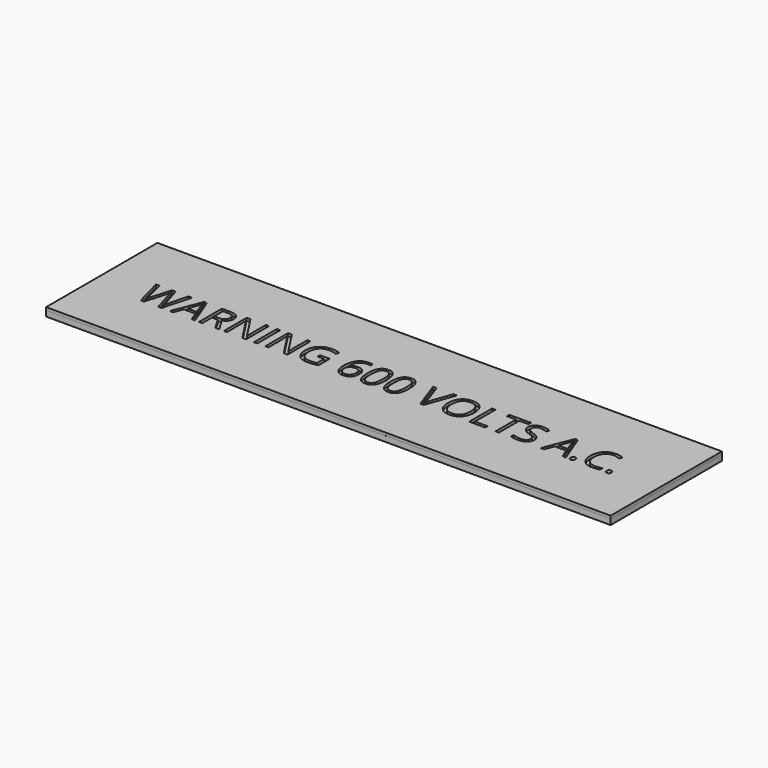
from build123d import *

# Parameters (mm, degrees)
F0_W         = 203.2
F0_H         = 50.08
F1_DEPTH     = 2
F2_DEPTH     = 1
F3_TEXT_SIZE = 14.4258524236
F4_DEPTH     = 1.1


# Not quite as in the source:
# - Text() gives the source's letters only with a copy of the font that has no kerning and outlines rounded to 1/6400 em; it was checked with that copy


with BuildPart() as f1:
    # F0 (on Top) → F1 (new body)
    with BuildSketch(Plane.XY):
        with Locations((75.894802174, 15.1347585702)):
            Rectangle(F0_W, F0_H)
    extrude(amount=F1_DEPTH)


with BuildPart() as f2:
    # F2 (new): a face of the model
    f2_faces = [f1.part.faces().sort_by_distance(p)[0] for p in [
        (75.894802174, 15.1347585702, 2),
    ]]
    extrude(f2_faces, amount=F2_DEPTH)

    # F3 (on face) → F4 (cut)
    with BuildSketch(Plane.XY.offset(3)):
        with Locations((-10.4268407449, 9.9412448252)):
            Text('WARNING 600 VOLTS A.C.', F3_TEXT_SIZE, font='Open Sans', text_align=(TextAlign.LEFT, TextAlign.BOTTOM))
    extrude(amount=-F4_DEPTH, mode=Mode.SUBTRACT)


solid = Compound([f1.part, f2.part])
